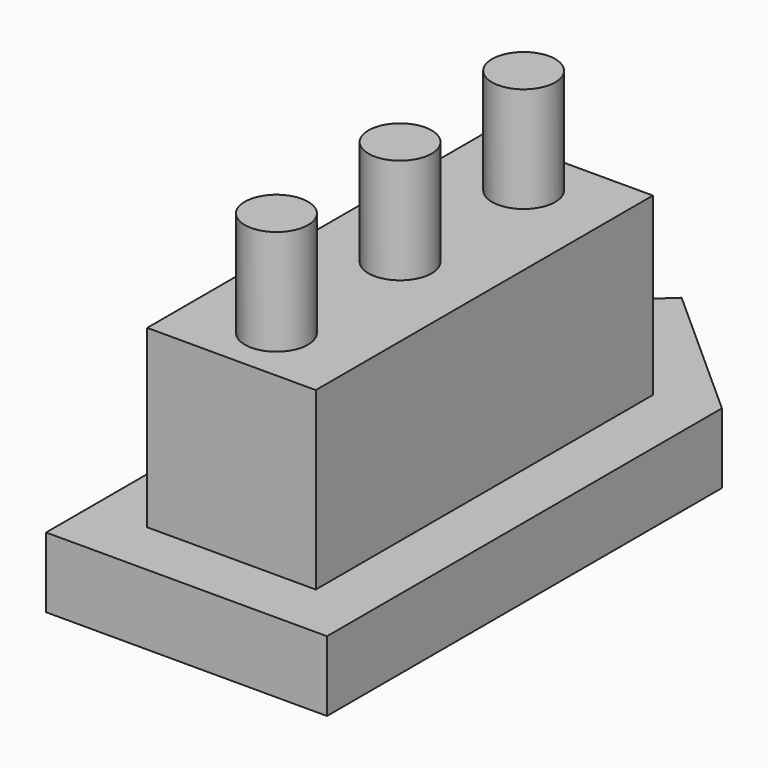
from build123d import *

# Parameters (mm, degrees)
F1_DEPTH     = 10
F2_W         = 24
F2_H         = 60
F3_DEPTH     = 25
F4_R         = 4.5
F5_DEPTH     = 15
F6_TEXT_SIZE = 15.2777777778
F7_DEPTH     = 5


# Not quite as in the source:
# - Text() gives the source's letters only with a copy of the font that has no kerning and outlines rounded to 1/6400 em; it was checked with that copy


with BuildPart() as f1:
    # F0 (on Top) → F1 (new body)
    with BuildSketch(Plane.XY):
        Polygon((-0.1311976347, 64.7275422611), (-20, 46.4455650002), (-20, -23.5544349998), (20, -23.5544349998), (20, 46.7349081629), align=None)
    extrude(amount=F1_DEPTH)

    # F2 (on face) → F3 (join)
    with BuildSketch(Plane.XY.offset(10)):
        with Locations((0, 14.4455650002)):
            Rectangle(F2_W, F2_H)
    extrude(amount=F3_DEPTH)

    # F4 (on face) → F5 (join)
    with BuildSketch(Plane.XY.offset(35)):
        with Locations((0, -7.5544349998)):
            Circle(F4_R)
        with Locations((0, 14.4455650002)):
            Circle(F4_R)
        with Locations((0, 36.4455650002)):
            Circle(F4_R)
    extrude(amount=F5_DEPTH)

    # F6 (on face) → F7 (cut)
    with BuildSketch(Plane(origin=(-12, 0, 0), x_dir=(0, -1, 0), z_dir=(-1, 0, 0))):
        with Locations((-35.0891668626, 17)):
            Text('Rahaf', F6_TEXT_SIZE, font='Open Sans', text_align=(TextAlign.LEFT, TextAlign.BOTTOM))
    extrude(amount=-F7_DEPTH, mode=Mode.SUBTRACT)


solid = f1.part
